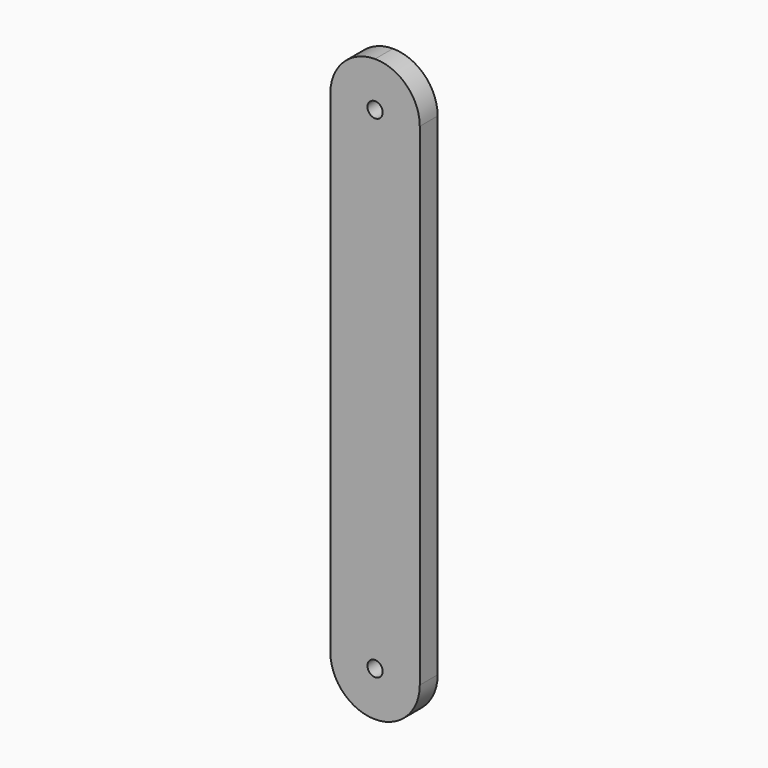
from build123d import *

# Parameters (mm, degrees)
F0_W     = 25.4
F0_H     = 165.1
F1_DEPTH = 6.35
F2_R     = 2.159
F3_DEPTH = 25.4
F4_R     = 12.69999


# Not quite as in the source:
# - a fillet or chamfer is up to 0.001 mm smaller than in the source, because OpenCascade refuses the exact size


with BuildPart() as f1:
    # F0 (on Front) → F1 (new body)
    with BuildSketch(Plane.XZ):
        with Locations((-124.4640206625, 27.955437386)):
            Rectangle(F0_W, F0_H)
    extrude(amount=F1_DEPTH)

    # F2 (on face) → F3 (cut)
    with BuildSketch(Plane.XZ.offset(6.35)):
        with Locations((-124.4640206625, 97.805437386)):
            Circle(F2_R)
        with Locations((-124.4640206625, -41.894562614)):
            Circle(F2_R)
    extrude(amount=-F3_DEPTH, mode=Mode.SUBTRACT)

    # F4 (radius 12.7 in the source; OpenCascade refuses exactly that, so slightly less here)
    f4_edges = [f1.edges().sort_by_distance(p)[0] for p in [
        (-137.164021, -3.175, 110.505437),
        (-111.764021, -3.175, 110.505437),
        (-137.164021, -3.175, -54.594563),
        (-111.764021, -3.175, -54.594563),
    ]]
    fillet(f4_edges, radius=F4_R)


solid = f1.part
